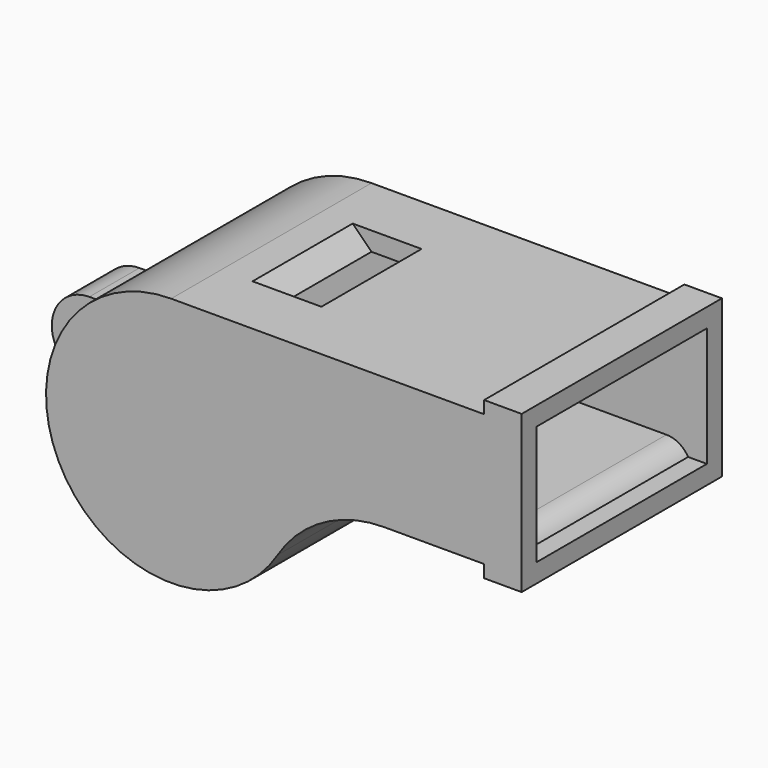
from build123d import *

# Parameters (mm, degrees)
F1_DEPTH    = 10
F2_T        = -1.5
F4_DEPTH    = 5
F5_R        = 1.75
F6_DEPTH    = 2.5
F9_T1_DEPTH = 17


# Not quite as in the source:
# - a fillet or chamfer that OpenCascade refuses, or shapes differently, is made with other operations: its cross-section is extruded or revolved along the edge and cut away or added


with BuildPart() as f1:
    # F0 (on Front) → F1 (new body, symmetric)
    with BuildSketch(Plane.XZ):
        with BuildLine():
            Line((25, 10), (0, 10))
            ThreePointArc((0, 10), (-8.7372269275, -4.8642435813), (8.5, -5.2678268764))
            ThreePointArc((8.5, -5.2678268764), (12.1357564187, -1.7984268254), (17, -0.5356537529))
            Line((17, -0.5356537529), (25, -0.5356537529))
            Line((25, -0.5356537529), (25, -1.5356537529))
            Line((25, -1.5356537529), (28, -1.5356537529))
            Line((28, -1.5356537529), (28, 11))
            Line((28, 11), (25, 11))
            Line((25, 11), (25, 10))
        make_face()
    extrude(amount=F1_DEPTH, both=True)

    # F2
    f2_openings = [f1.faces().sort_by_distance(p)[0] for p in [
        (28, 0, 4.732173),
    ]]
    offset(amount=F2_T, openings=f2_openings, kind=Kind.INTERSECTION)

    # F3 (on Front) → F4 (cut, symmetric)
    with BuildSketch(Plane.XZ):
        Polygon((8, 10), (2.5, 10), (4, 8.5), (6.5, 8.5), align=None)
    extrude(amount=F4_DEPTH, both=True, mode=Mode.SUBTRACT)

    # F5 (on Front) → F6 (join, symmetric)
    with BuildSketch(Plane.XZ):
        with BuildLine():
            Line((-9.5393920142, 3), (-12.5393920142, 3))
            ThreePointArc((-12.5393920142, 3), (-15.5393920142, 0), (-12.5393920142, -3))
            Line((-12.5393920142, -3), (-9.5393920142, -3))
            Line((-9.5393920142, -3), (-9.5393920142, 3))
        make_face()
        with Locations((-12.5393920142, 0)):
            Circle(F5_R, mode=Mode.SUBTRACT)
    extrude(amount=F6_DEPTH, both=True)

    # F9: fillet of radius 2 on 2 edges, made by hand

    # F9_s2 → F9_t1 (cut)
    with BuildSketch(Plane.XZ.offset(-8.5)):
        with BuildLine():
            ThreePointArc((24.7679491924, 0.9643462471), (25.7679491924, 0.6963970547), (26.5, -0.0356537529))
            Line((26.5, -0.0356537529), (26.5, 0.9643462471))
            Line((26.5, 0.9643462471), (24.7679491924, 0.9643462471))
        make_face()
        with BuildLine():
            ThreePointArc((24.7679491924, 8.5), (25.7679491924, 8.7679491924), (26.5, 9.5))
            Line((26.5, 9.5), (26.5, 8.5))
            Line((26.5, 8.5), (24.7679491924, 8.5))
        make_face()
    extrude(amount=F9_T1_DEPTH, mode=Mode.SUBTRACT)


with BuildPart() as f8:
    # F7 (on Front) → F8 (revolve)
    with BuildSketch(Plane.XZ):
        with BuildLine():
            Line((0, 1.5), (0, -8.5))
            ThreePointArc((0, -8.5), (5, -3.5), (0, 1.5))
        make_face()
    revolve(axis=Axis((0, 0, -3.5), (0, 0, -1)))


solid = Compound([f1.part, f8.part])
